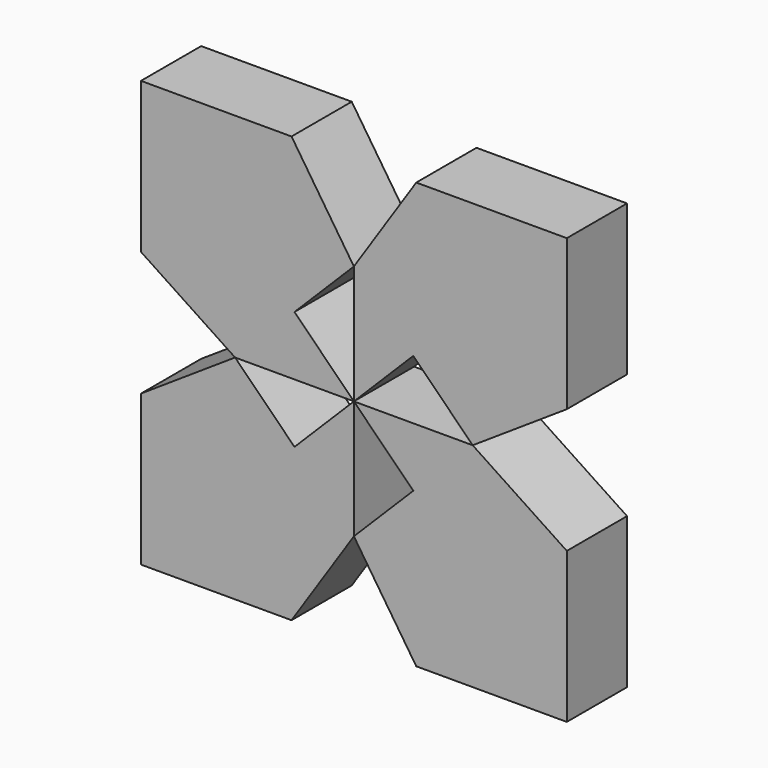
from build123d import *

# Parameters (mm, degrees)
F2_DEPTH = 25.4


# Not quite as in the source:
# - a feature of the source that left no trace in its solid (it failed there, or was rolled back) is left out


with BuildPart() as f2:
    # F0 (on Front) → F2 (new body)
    with BuildSketch(Plane.XZ):
        Polygon((0, 40.0797729921), (20.039886496, 20.039886496), (71.8420489686, 71.8420489686), (21.0420489686, 71.8420489686), align=None)
        Polygon((71.8420489686, 71.8420489686), (20.039886496, 20.039886496), (40.0797729921, 0), (71.8420489686, 21.0420489686), align=None)
        Polygon((0, 40.0797729921), (0, 0), (20.039886496, 20.039886496), align=None)
    extrude(amount=F2_DEPTH)


with BuildPart() as f2b:
    # F0 (on Front) → F2, piece 2 (new body)
    with BuildSketch(Plane.XZ):
        Polygon((71.8420489686, -71.8420489686), (20.039886496, -20.039886496), (0, -40.0797729921), (21.0420489686, -71.8420489686), align=None)
        Polygon((40.0797729921, 0), (20.039886496, -20.039886496), (71.8420489686, -71.8420489686), (71.8420489686, -21.0420489686), align=None)
        Polygon((40.0797729921, 0), (0, 0), (20.039886496, -20.039886496), align=None)
    extrude(amount=F2_DEPTH)


with BuildPart() as f2c:
    # F0 (on Front) → F2, piece 3 (new body)
    with BuildSketch(Plane.XZ):
        Polygon((-71.8420489686, -71.8420489686), (-20.039886496, -20.039886496), (-40.0797729921, 0), (-71.8420489686, -21.0420489686), align=None)
        Polygon((0, -40.0797729921), (-20.039886496, -20.039886496), (-71.8420489686, -71.8420489686), (-21.0420489686, -71.8420489686), align=None)
        Polygon((0, -40.0797729921), (0, 0), (-20.039886496, -20.039886496), align=None)
    extrude(amount=F2_DEPTH)


with BuildPart() as f2d:
    # F0 (on Front) → F2, piece 4 (new body)
    with BuildSketch(Plane.XZ):
        Polygon((-71.8420489686, 71.8420489686), (-20.039886496, 20.039886496), (0, 40.0797729921), (-21.0420489686, 71.8420489686), align=None)
        Polygon((-40.0797729921, 0), (-20.039886496, 20.039886496), (-71.8420489686, 71.8420489686), (-71.8420489686, 21.0420489686), align=None)
        Polygon((-40.0797729921, 0), (0, 0), (-20.039886496, 20.039886496), align=None)
    extrude(amount=F2_DEPTH)


solid = Compound([f2.part, f2b.part, f2c.part, f2d.part])
